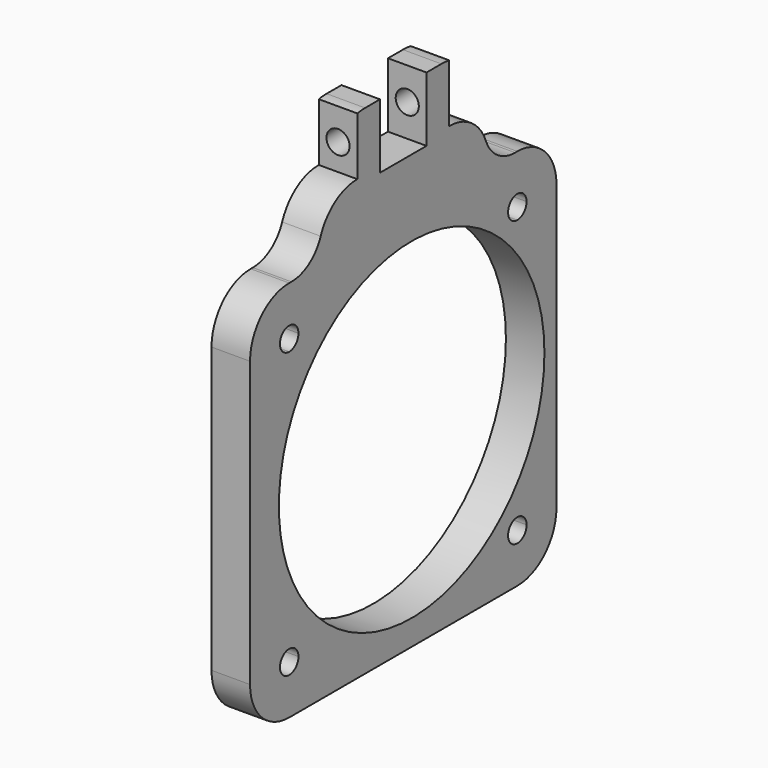
from build123d import *

# Parameters (mm, degrees)
F1_DEPTH       = 5
F2_R           = 21.536165151
F3_DEPTH       = 5.001
F4_W           = 5
F4_H           = 27.6149739623
F5_DEPTH       = 15
F6_R           = 7.62
F7_W           = 5
F7_H           = 7.544119532
F8_DEPTH       = 8.382
F9_R           = 1.5
F10_DEPTH      = 21.078940234
F10_DEPTH_BACK = 28.623059766
F11_W          = 7.3633623496
F11_H          = 12.0904415441
F12_DEPTH      = 6.35
F13_W          = 7.1302087698
F13_H          = 20.9519683909
F14_DEPTH      = 6.35
F15_R          = 6.34999
F16_R          = 5.08


# Not quite as in the source:
# - a fillet or chamfer is up to 0.001 mm smaller than in the source, because OpenCascade refuses the exact size


with BuildPart() as f1:
    # F0 (on Right) → F1 (new body)
    with BuildSketch(Plane.YZ):
        with BuildLine():
            ThreePointArc((0, 6.35), (-4.4901280605, 4.4901280605), (-6.35, 0))
            Line((-6.35, 0), (-6.35, -36.927669698))
            ThreePointArc((-6.35, -36.927669698), (-4.4901280605, -41.4177977585), (0, -43.277669698))
            Line((0, -43.277669698), (37, -43.277669698))
            ThreePointArc((37, -43.277669698), (41.4901280605, -41.4177977585), (43.35, -36.927669698))
            Line((43.35, -36.927669698), (43.35, 0))
            ThreePointArc((43.35, 0), (41.4901280605, 4.4901280605), (37, 6.35))
            Line((37, 6.35), (0, 6.35))
        make_face()
        with BuildLine():
            ThreePointArc((0, -1.5), (-1.0606601718, 1.0606601718), (1.5, 0))
            Line((1.5, 0), (35.5, 0))
            ThreePointArc((35.5, 0), (37, 1.5), (38.5, 0))
            ThreePointArc((38.5, 0), (38.0606601718, -1.0606601718), (37, -1.5))
            Line((37, -1.5), (37, -35.4276701232))
            ThreePointArc((37, -35.4276701232), (38.0606601718, -35.8670099514), (38.5, -36.9276701232))
            ThreePointArc((38.5, -36.9276701232), (37, -38.4276701232), (35.5, -36.9276701232))
            Line((35.5, -36.9276701232), (1.5, -36.9276701232))
            ThreePointArc((1.5, -36.9276701232), (-1.0606601718, -37.988330295), (0, -35.4276701232))
            Line((0, -35.4276701232), (0, -1.5))
        make_face(mode=Mode.SUBTRACT)
        with BuildLine():
            Line((35.5, 0), (1.5, 0))
            ThreePointArc((1.5, 0), (1.0606601718, -1.0606601718), (0, -1.5))
            Line((0, -1.5), (0, -35.4276701232))
            ThreePointArc((0, -35.4276701232), (1.0606601718, -35.8670099514), (1.5, -36.9276701232))
            Line((1.5, -36.9276701232), (35.5, -36.9276701232))
            ThreePointArc((35.5, -36.9276701232), (35.9393398282, -35.8670099514), (37, -35.4276701232))
            Line((37, -35.4276701232), (37, -1.5))
            ThreePointArc((37, -1.5), (35.9393398282, -1.0606601718), (35.5, 0))
        make_face()
    extrude(amount=F1_DEPTH)

    # F2 (on face) → F3 (cut, through all)
    with BuildSketch(Plane.YZ.offset(5)):
        with Locations((19.8611337692, -18.463834849)):
            Circle(F2_R)
    extrude(amount=-F3_DEPTH, mode=Mode.SUBTRACT)

    # F4 (on face) → F5 (join)
    with BuildSketch(Plane.XY.offset(6.35)):
        with Locations((2.5, 18.5)):
            Rectangle(F4_W, F4_H)
    extrude(amount=F5_DEPTH)

    # F6
    f6_edges = [f1.edges().sort_by_distance(p)[0] for p in [
        (2.5, 32.307487, 21.35),
        (2.5, 4.692513, 21.35),
    ]]
    fillet(f6_edges, radius=F6_R)

    # F7 (on face) → F8 (cut)
    with BuildSketch(Plane.XY.offset(21.35)):
        with Locations((2.5, 18.5)):
            Rectangle(F7_W, F7_H)
    extrude(amount=-F8_DEPTH, mode=Mode.SUBTRACT)

    # F9 (on face) → F10 (cut, two sides)
    with BuildSketch(Plane(origin=(0, 14.727940234, 0), x_dir=(-1, 0, 0), z_dir=(0, 1, 0))) as f10_sk:
        with Locations((-2.5, 17.159)):
            Circle(F9_R)
    extrude(amount=-F10_DEPTH, mode=Mode.SUBTRACT)
    extrude(f10_sk.sketch, amount=F10_DEPTH_BACK, mode=Mode.SUBTRACT)

    # F11 (on face) → F12 (cut)
    with BuildSketch(Plane(origin=(0, 32.3074869812, 0), x_dir=(-1, 0, 0), z_dir=(0, 1, 0))):
        with Locations((-1.3183188252, 19.775220772)):
            Rectangle(F11_W, F11_H)
    extrude(amount=-F12_DEPTH, mode=Mode.SUBTRACT)

    # F13 (on face) → F14 (cut)
    with BuildSketch(Plane.XZ.offset(-4.6925130188)):
        with Locations((1.4348956151, 24.2059841955)):
            Rectangle(F13_W, F13_H)
    extrude(amount=-F14_DEPTH, mode=Mode.SUBTRACT)

    # F15 (radius 6.35 in the source; OpenCascade refuses exactly that, so slightly less here)
    f15_edges = [f1.edges().sort_by_distance(p)[0] for p in [
        (2.5, 4.692513, 13.73),
        (2.5, 32.307487, 13.73),
    ]]
    fillet(f15_edges, radius=F15_R)

    # F16
    f16_edges = [f1.edges().sort_by_distance(p)[0] for p in [
        (2.5, 4.692513, 6.35),
        (2.5, 32.307487, 6.35),
    ]]
    fillet(f16_edges, radius=F16_R)


solid = f1.part
